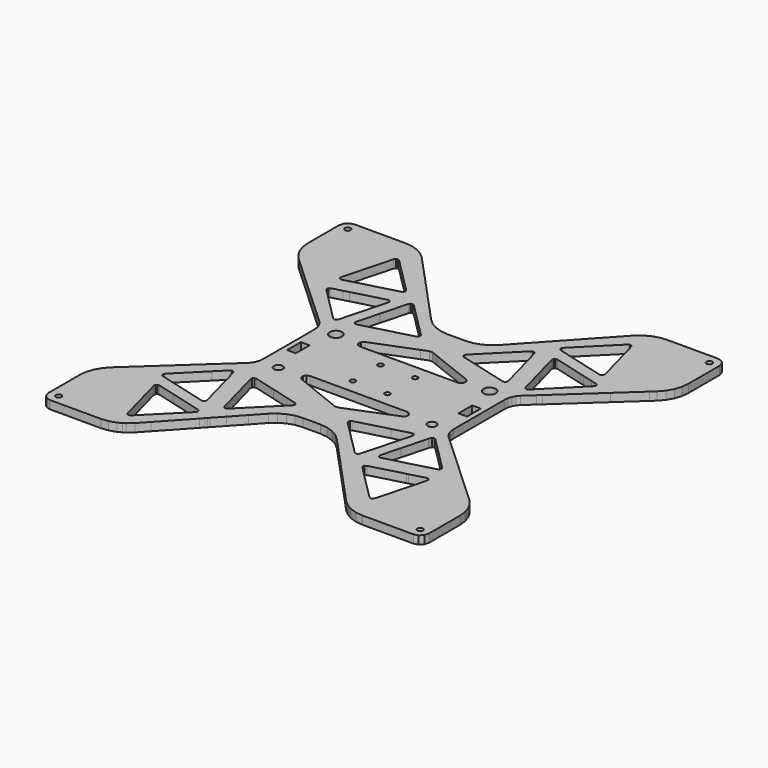
from build123d import *

# Parameters (mm, degrees)
F0_W     = 5.000752
F0_H     = 9.997694
F0_W_2   = 4.999482
F1_DEPTH = 4.75
F2_R     = 1.525
F2_R_2   = 1.65
F2_R_3   = 3.555
F2_R_4   = 2.55
F3_DEPTH = 4.751


# Not quite as in the source:
# - a pattern or mirror of a feature is missing from the dataset's text; its kind, count and spacing are read off the source's solid


with BuildPart() as f1:
    # F0 (on Top) → F1 (new body)
    with BuildSketch(Plane.XY):
        Polygon((109.9695794, -105.1112452), (109.9998054, -105.0010092), (109.9998054, -82.5113158), (109.5753714, -78.4104858), (108.3175634, -74.4813598), (106.2820074, -70.8958958), (103.5550634, -67.8036998), (101.0922794, -65.5352258), (81.7224934, -47.6802958), (75.0019074, -41.4829498), (66.2899614, -33.4519778), (65.5360894, -32.7588118), (58.2216514, -26.0146038), (56.8571634, -24.4712998), (55.8404014, -22.6770438), (55.2117514, -20.7118458), (54.9996614, -18.6640978), (54.9996614, 18.6670442), (55.2117514, 20.7160622), (55.8404014, 22.6810062), (56.8571634, 24.4737382), (58.2216514, 26.0200902), (63.4027434, 30.7947822), (65.5360894, 32.7602342), (88.1210074, 53.5793442), (101.0922794, 65.5369022), (103.5550634, 67.8076622), (106.2820074, 70.8985882), (108.3175634, 74.4843062), (109.5753714, 78.4116542), (109.9998054, 82.5127382), (109.9998054, 105.0024062), (109.9751674, 105.1266122), (109.6180434, 106.9165502), (108.5349874, 108.5396102), (107.9794894, 108.9091802), (106.9129434, 109.6244442), (105.0003234, 110.0018882), (75.7103134, 110.0018882), (71.6092294, 109.5789782), (67.6816274, 108.3206622), (65.5360894, 107.1024782), (64.0961634, 106.2868842), (61.0037134, 103.5581622), (44.9991734, 86.1975162), (34.4571574, 74.7598962), (25.9562854, 65.5369022), (19.7673214, 58.8216502), (16.6748714, 56.0944522), (13.0894074, 54.0576262), (9.1633294, 52.8021042), (5.0622454, 52.3764002), (-5.0621946, 52.3764002), (-9.1632786, 52.8021042), (-13.0906266, 54.0576262), (-16.6748206, 56.0944522), (-19.7672706, 58.8216502), (-25.9575046, 65.5369022), (-34.8096586, 75.1414042), (-42.3039286, 83.2706742), (-43.9531506, 85.0595962), (-59.3971126, 101.8149602), (-61.0034086, 103.5581622), (-64.0958586, 106.2868842), (-65.5360386, 107.1024782), (-67.6815766, 108.3206622), (-71.6091786, 109.5789782), (-75.7100086, 110.0018882), (-105.000298, 110.0018882), (-105.1146488, 109.9716622), (-107.500039, 109.3348842), (-108.8711818, 107.9625222), (-109.3300836, 107.5022742), (-109.9681062, 105.1222942), (-109.9998054, 105.0024062), (-109.9998054, 82.5127382), (-109.5753714, 78.4116542), (-108.3186048, 74.4843062), (-106.281855, 70.8985882), (-103.5547078, 67.8076622), (-101.0921778, 65.5369022), (-75.4428006, 41.8922962), (-66.2624786, 33.4297782), (-65.5360386, 32.7602342), (-58.2228706, 26.0200902), (-56.8583826, 24.4737382), (-55.8416206, 22.6810062), (-55.2117006, 20.7160622), (-55.0011346, 18.6670442), (-55.0011346, -18.6640978), (-55.2117006, -20.7118458), (-55.8416206, -22.6770438), (-56.8583826, -24.4712998), (-58.2228706, -26.0146038), (-65.5360386, -32.7588118), (-91.6291538, -56.8098178), (-101.0921778, -65.5352258), (-103.5547078, -67.8036998), (-106.281855, -70.8958958), (-108.3186048, -74.4813598), (-109.5753714, -78.4104858), (-109.9998054, -82.5113158), (-109.9998054, -105.0010092), (-109.6194658, -106.9151024), (-108.534962, -108.5356732), (-106.9130196, -109.620177), (-105.000298, -110.0018882), (-75.7100086, -110.0018882), (-71.6091786, -109.5760826), (-67.6815766, -108.317919), (-65.5360386, -107.1025036), (-64.0958586, -106.2853094), (-61.0034086, -103.555419), (-56.1626766, -98.303715), (-41.0593286, -81.9187338), (-39.4210286, -80.1397178), (-38.6229606, -79.2743398), (-37.7712986, -78.3510498), (-32.7674986, -72.9228158), (-25.9575046, -65.5352258), (-19.7672706, -58.8202278), (-16.6748206, -56.0917598), (-13.0906266, -54.0562038), (-9.1632786, -52.7996658), (-5.0621946, -52.3734538), (5.0622454, -52.3734538), (9.1633294, -52.7996658), (13.0894074, -54.0562038), (16.6748714, -56.0917598), (19.7673214, -58.8202278), (20.4302614, -59.5395558), (25.9575554, -65.5352258), (37.1015514, -77.6248638), (42.6649134, -83.6606658), (59.4284054, -101.8466594), (60.0181934, -102.4874506), (61.0037134, -103.555419), (64.0961634, -106.2853094), (65.5360894, -107.1025036), (67.6816274, -108.317919), (71.6092294, -109.5760826), (75.7103134, -110.0018882), (105.0003234, -110.0018882), (105.1120834, -109.971586), (107.4999374, -109.3307948), (109.3302614, -107.5021218), align=None)
        Polygon((-46.6112606, -75.8486418), (-46.1715866, -76.1559818), (-45.9056486, -77.1481058), (-46.3399886, -78.0782538), (-49.1527846, -80.8895258), (-50.1807226, -81.9187338), (-66.5639766, -98.303715), (-67.1606226, -98.8976686), (-68.0907706, -99.3331262), (-69.0818786, -99.0671628), (-69.6147706, -98.303715), (-69.6701426, -98.2252036), (-77.2906506, -69.7851538), (-77.2009886, -68.7615338), (-76.4763266, -68.0366178), (-75.4537226, -67.9469558), (-65.5360386, -70.6050658), (-49.1527846, -74.9944398), (-47.0123266, -75.5677178), align=None, mode=Mode.SUBTRACT)
        Polygon((-59.8004646, -36.6117378), (-58.8715866, -36.1761278), (-57.8797166, -36.4407958), (-57.8146926, -36.5345218), (-57.2911986, -37.2840758), (-55.3770546, -44.4250318), (-49.7420646, -65.4557238), (-49.7217446, -65.5352258), (-49.6704366, -65.7254718), (-49.7600986, -66.7468058), (-50.4850146, -67.4727378), (-51.5073646, -67.5639238), (-59.0745326, -65.5352258), (-65.5360386, -63.8044698), (-79.9490146, -59.9406218), (-80.7895006, -59.3521038), (-81.0554386, -58.3612498), (-80.6213526, -57.4298318), (-65.5360386, -42.3457878), align=None, mode=Mode.SUBTRACT)
        Polygon((-32.7674986, -38.8456678), (-17.0123866, -43.0651158), (-16.1719006, -43.6549038), (-15.9059626, -44.6470278), (-16.3400486, -45.5771758), (-32.7674986, -62.0061498), (-36.2980986, -65.5352258), (-37.1606826, -66.3965398), (-38.0910846, -66.8321498), (-39.0819386, -66.5662118), (-39.6704566, -65.7254718), (-39.7212566, -65.5352258), (-47.2907106, -37.2840758), (-47.2025726, -36.2604558), (-46.4763866, -35.5368098), (-45.4537826, -35.4471478), align=None, mode=Mode.SUBTRACT)
        Polygon((66.5157674, -65.5352258), (75.2345714, -63.1996958), (76.2574294, -63.2891038), (76.9818374, -64.0127498), (77.0714994, -65.0378938), (76.9378954, -65.5352258), (69.4512454, -93.4792136), (68.8614574, -94.3184296), (67.8703494, -94.584393), (66.9402014, -94.1489608), (46.1208374, -73.3309938), (45.6867514, -72.4008458), (45.9526894, -71.4087218), (46.7934294, -70.8189338), (65.5360894, -65.7986238), align=None, mode=Mode.SUBTRACT)
        Polygon((13.6212834, -43.3297838), (13.1869434, -42.3993818), (13.4531354, -41.4075118), (14.2923514, -40.8189938), (32.7675494, -35.8675178), (42.7350174, -33.1982318), (43.7563514, -33.2878938), (44.4822834, -34.0128098), (44.5719454, -35.0366838), (36.9501674, -63.4793498), (36.3631734, -64.3185658), (35.3707954, -64.5832338), (34.4419174, -64.1488938), align=None, mode=Mode.SUBTRACT)
        Polygon((30.6126134, -20.3232258), (30.3492154, -22.0199458), (29.0677854, -23.1621838), (5.2154074, -32.7654158), (3.6771834, -33.3869538), (1.0109454, -34.4606118), (-0.0004826, -34.4606118), (-0.8838946, -34.4618818), (-3.9819326, -33.2177898), (-5.1061366, -32.7654158), (-29.0443666, -23.1634538), (-30.3283366, -22.0237558), (-30.5917346, -20.3260198), (-29.7154346, -18.8487558), (-28.0989786, -18.2673498), (28.1183334, -18.2673498), (29.7347894, -18.8487558), align=None, mode=Mode.SUBTRACT)
        Polygon((74.9231674, -51.9988038), (74.6584994, -52.9883878), (73.8182674, -53.5781758), (68.0842174, -55.1161458), (65.5360894, -55.7968658), (46.7934294, -60.8197158), (45.7710794, -60.7315778), (45.0461634, -60.0038678), (44.9549774, -58.9827878), (47.9689414, -47.7394778), (51.9803634, -32.7654158), (52.1965174, -31.9564258), (52.7850354, -31.1146698), (53.7774134, -30.8502558), (54.7060374, -31.2840878), (54.9996614, -31.5777118), (56.1904134, -32.7654158), (57.5185794, -34.0968838), (74.4906054, -51.0686558), align=None, mode=Mode.SUBTRACT)
        Polygon((-52.7890486, 32.7683622), (-53.2576786, 32.1016122), (-54.2500566, 31.8341502), (-55.1789346, 32.2667122), (-55.6800766, 32.7683622), (-65.5360386, 42.6266102), (-74.9619786, 52.0525502), (-75.3958106, 52.9814282), (-75.1298726, 53.9748222), (-74.2906566, 54.5633402), (-68.5553366, 56.0985162), (-65.5360386, 56.9075062), (-47.2645486, 61.8036102), (-46.2432146, 61.7126782), (-45.5172826, 60.9890322), (-45.4276206, 59.9654122), (-48.3257606, 49.1531402), (-52.6691606, 32.9418442), align=None, mode=Mode.SUBTRACT)
        with Locations((-49.5005106, 0.0019812)):
            Rectangle(F0_W, F0_H, mode=Mode.SUBTRACT)
        Polygon((-30.7997606, 22.0404182), (-29.5043606, 23.1760522), (-5.1005486, 32.7683622), (-1.2285726, 34.2913462), (0.6291834, 34.2913462), (4.5014134, 32.7683622), (28.9049714, 23.1760522), (30.2003714, 22.0404182), (30.4716434, 20.3414122), (29.5968674, 18.8572902), (27.9760934, 18.2741062), (-28.5754826, 18.2741062), (-30.1947326, 18.8572902), (-31.0712866, 20.3414122), align=None, mode=Mode.SUBTRACT)
        Polygon((-32.7674986, 36.9784122), (-43.2061366, 34.1808562), (-44.2289946, 34.2717882), (-44.9536566, 34.9979742), (-45.0445886, 36.0177842), (-41.5249106, 49.1531402), (-37.4294146, 64.4411462), (-37.4228106, 64.4604502), (-36.8342926, 65.3011902), (-35.9549446, 65.5369022), (-35.8434386, 65.5656042), (-35.7784146, 65.5369022), (-34.9130366, 65.1343122), (-34.8980506, 65.1190722), (-32.7674986, 62.9887742), (-14.0939266, 44.3121542), (-13.6595866, 43.3820062), (-13.9242546, 42.3924222), (-14.7649946, 41.8039042), align=None, mode=Mode.SUBTRACT)
        Polygon((-70.6526146, 65.5369022), (-75.7059446, 64.1820662), (-76.7285486, 64.2717282), (-77.4547346, 64.9991842), (-77.5014706, 65.5369022), (-77.5428726, 66.0189942), (-69.9236346, 94.4616602), (-69.3341006, 95.3011302), (-68.3429926, 95.5670682), (-67.4128446, 95.1342522), (-46.5922106, 74.3120942), (-46.1593946, 73.3819462), (-46.4240626, 72.3923622), (-47.2645486, 71.8043522), (-48.5188006, 71.4690722), (-65.5360386, 66.9095182), align=None, mode=Mode.SUBTRACT)
        with Locations((49.4999264, 0.0019812)):
            Rectangle(F0_W_2, F0_H, mode=Mode.SUBTRACT)
        Polygon((32.7675494, 34.6743782), (14.5458434, 39.5565122), (13.7053574, 40.1450302), (13.4391654, 41.1343602), (13.8735054, 42.0647622), (34.6941394, 62.8853962), (35.6245414, 63.3194822), (36.6153954, 63.0535442), (37.2034054, 62.2128042), (40.7022554, 49.1531402), (44.8241674, 33.7716622), (44.7360294, 32.7683622), (44.7345054, 32.7503282), (44.0095894, 32.0228722), (42.9872394, 31.9347342), (39.8742154, 32.7683622), align=None, mode=Mode.SUBTRACT)
        Polygon((77.4822174, 56.4304942), (78.3229574, 55.8422302), (78.5873714, 54.8485822), (78.1550634, 53.9197042), (65.5360894, 41.2999682), (57.3339214, 33.0978002), (56.6242454, 32.7683622), (56.4037734, 32.6649842), (56.0182014, 32.7683622), (55.4131734, 32.9309222), (54.8233854, 33.7716622), (50.7027434, 49.1531402), (47.2038934, 62.2128042), (47.2922854, 63.2366782), (48.0184714, 63.9615942), (49.0408214, 64.0497322), (65.5360894, 59.6319102), (68.3526954, 58.8752442), (74.0468674, 57.3499742), align=None, mode=Mode.SUBTRACT)
        Polygon((68.8736494, 65.5369022), (65.5360894, 66.4309822), (44.5457834, 72.0560662), (43.7050434, 72.6458542), (43.4391054, 73.6354382), (43.8734454, 74.5671102), (64.6940794, 95.3864742), (65.5360894, 95.7804282), (65.6242274, 95.8220842), (66.6153354, 95.5546222), (67.2035994, 94.7138822), (74.8241074, 66.2712162), (74.7593374, 65.5369022), (74.7344454, 65.2498822), (74.0085134, 64.5239502), (72.9871794, 64.4342882), align=None, mode=Mode.SUBTRACT)
    extrude(amount=F1_DEPTH)

    # F2 (on face) → F3 (cut, through all)
    with BuildSketch(Plane.XY.offset(4.75)):
        with Locations((-10, 10)):
            Circle(F2_R)
        with Locations((-10, -10)):
            Circle(F2_R)
        with Locations((-104.5, 104.5)):
            Circle(F2_R_2)
        with Locations((-104.5, -104.5)):
            Circle(F2_R_2)
        with Locations((-44.445, 20.8)):
            Circle(F2_R_3)
        with Locations((-44.445, -20.8)):
            Circle(F2_R_4)
    f3 = extrude(amount=-F3_DEPTH, mode=Mode.SUBTRACT)

    # F3_copies: F3 across plane
    add(f3.mirror(Plane(origin=(0, 0, 0), x_dir=(0, 0, 1), z_dir=(1, 0, 0))), mode=Mode.SUBTRACT)


solid = f1.part
